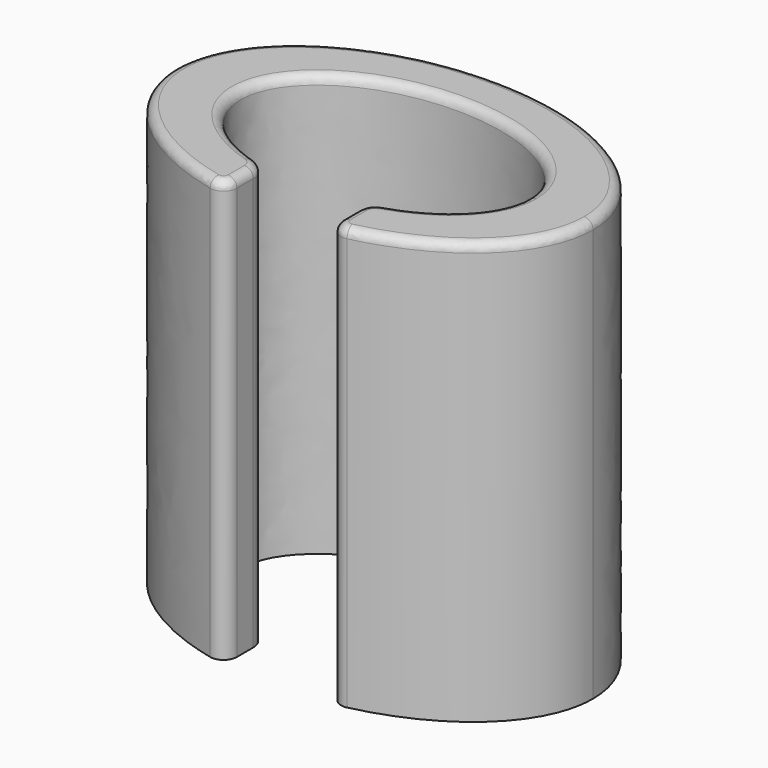
from build123d import *

# Parameters (mm, degrees)
F2_DEPTH = 12.1
F3_W     = 2.9972
F3_H     = 7.8756082803
F4_DEPTH = 25.4
F5_R     = 0.508
F6_R     = 0.381
F7_R     = 0.254


with BuildPart() as f2:
    # F0 (on Top) → F2 (new body)
    with BuildSketch(Plane.XY):
        with BuildLine():
            add(Edge.make_bspline(
                [(6, 0), (6, 6.9282032303), (-3, 3.4641016151), (-12, 0), (-3, -3.4641016151), (6, -6.9282032303), (6, 0)],
                knots=[0, 0, 0, 2.0943951024, 2.0943951024, 4.1887902048, 4.1887902048, 6.2831853072, 6.2831853072, 6.2831853072], degree=2, weights=[1, 0.5, 1, 0.5, 1, 0.5, 1]))
        make_face()
        with BuildLine():
            add(Edge.make_bspline(
                [(4.115, 0), (4.115, 4.5293128618), (-2.0575, 2.2646564309), (-8.23, 0), (-2.0575, -2.2646564309), (4.115, -4.5293128618), (4.115, 0)],
                knots=[0, 0, 0, 2.0943951024, 2.0943951024, 4.1887902048, 4.1887902048, 6.2831853072, 6.2831853072, 6.2831853072], degree=2, weights=[1, 0.5, 1, 0.5, 1, 0.5, 1]))
        make_face(mode=Mode.SUBTRACT)
    extrude(amount=F2_DEPTH)

    # F3 (on Top) → F4 (cut)
    with BuildSketch(Plane.XY):
        with Locations((0, -3.9378041402)):
            Rectangle(F3_W, F3_H)
    extrude(amount=F4_DEPTH, mode=Mode.SUBTRACT)

    # F5
    f5_edges = [f2.edges().sort_by_distance(p)[0] for p in [
        (1.4986, -2.435424, 6.05),
        (-1.4986, -2.435424, 6.05),
    ]]
    fillet(f5_edges, radius=F5_R)

    # F6
    f6_edges = [f2.edges().sort_by_distance(p)[0] for p in [
        (1.4986, -3.873224, 6.05),
        (-1.4986, -3.873224, 6.05),
    ]]
    fillet(f6_edges, radius=F6_R)

    # F7
    f7_edges = [f2.edges().sort_by_distance(p)[0] for p in [
        (-1.713626, 2.377469, 12.1),
        (-2.916698, 3.495576, 12.1),
        (-1.596258, -2.519622, 12.1),
        (-1.4986, -3.113596, 12.1),
        (-1.642459, -3.706302, 12.1),
        (1.642459, -3.706302, 12.1),
        (1.4986, -3.113596, 12.1),
        (1.596258, -2.519622, 12.1),
    ]]
    fillet(f7_edges, radius=F7_R)


solid = f2.part
